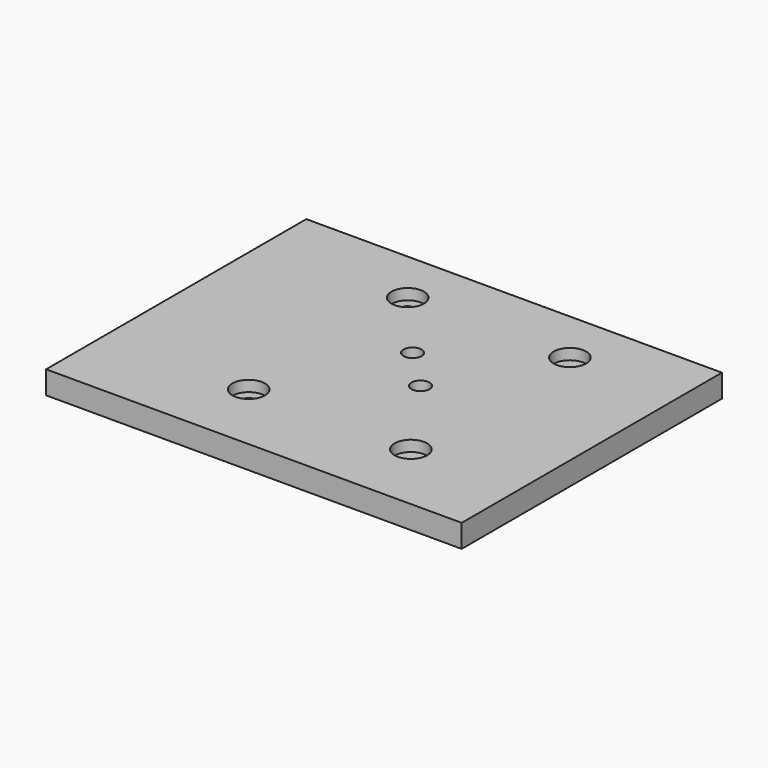
from build123d import *

# Parameters (mm, degrees)
F0_W     = 230
F0_H     = 180
F0_R     = 3.56
F0_R_2   = 2.5
F1_DEPTH = 12.7
F2_R     = 9
F2_R_2   = 5
F3_DEPTH = 6


# Not quite as in the source:
# - a length typed as a fraction of an inch, garbled in the dataset ("3 / 203.2 mm" for 3/8 in), is restored


with BuildPart() as f1:
    # F0 (on Top) → F1 (new body)
    with BuildSketch(Plane.XY):
        Rectangle(F0_W, F0_H)
        with Locations((-34.875, -50)):
            Circle(F0_R, mode=Mode.SUBTRACT)
        with Locations((54.875, -50)):
            Circle(F0_R_2, mode=Mode.SUBTRACT)
        with Locations((21, -1)):
            Circle(F0_R_2, mode=Mode.SUBTRACT)
        with Locations((-1, 21)):
            Circle(F0_R_2, mode=Mode.SUBTRACT)
        with Locations((-34.875, 60)):
            Circle(F0_R, mode=Mode.SUBTRACT)
        with Locations((54.875, 60)):
            Circle(F0_R_2, mode=Mode.SUBTRACT)
    extrude(amount=F1_DEPTH)

    # F2 (on face) → F3 (cut)
    with BuildSketch(Plane.XY.offset(12.7)):
        with Locations((-34.875, 60)):
            Circle(F2_R)
        with Locations((54.875, 60)):
            Circle(F2_R)
        with Locations((-34.875, -50)):
            Circle(F2_R)
        with Locations((54.875, -50)):
            Circle(F2_R)
        with Locations((-1, 21)):
            Circle(F2_R_2)
        with Locations((21, -1)):
            Circle(F2_R_2)
    extrude(amount=-F3_DEPTH, mode=Mode.SUBTRACT)


solid = f1.part
